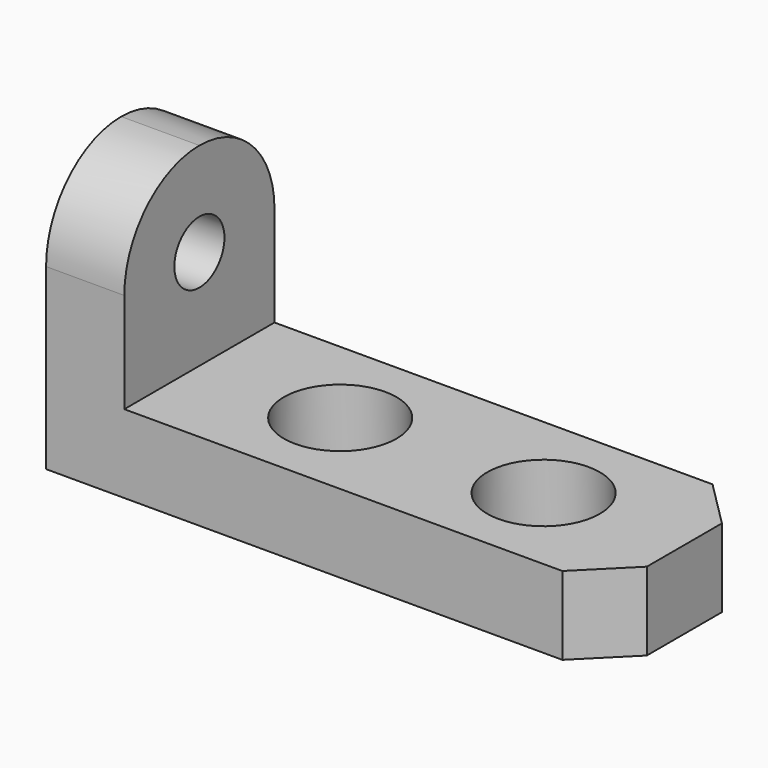
from build123d import *

# Parameters (mm, degrees)
F0_W     = 4572
F0_H     = 1524
F1_DEPTH = 635
F2_W     = 635
F2_H     = 1524
F3_DEPTH = 1574.8
F4_R     = 761.99999
F5_R     = 457.2
F6_DEPTH = 2540
F7_R     = 254
F8_DEPTH = 635
F9_SIZE  = 381


# Not quite as in the source:
# - a fillet or chamfer is up to 0.001 mm smaller than in the source, because OpenCascade refuses the exact size


with BuildPart() as f1:
    # F0 (on Top) → F1 (new body)
    with BuildSketch(Plane.XY):
        with Locations((2286, 762)):
            Rectangle(F0_W, F0_H)
    extrude(amount=F1_DEPTH)

    # F2 (on face) → F3 (join)
    with BuildSketch(Plane.XY.offset(635)):
        with Locations((317.5, 762)):
            Rectangle(F2_W, F2_H)
    extrude(amount=F3_DEPTH)

    # F4 (radius 762 in the source; OpenCascade refuses exactly that, so slightly less here)
    f4_edges = [f1.edges().sort_by_distance(p)[0] for p in [
        (317.5, 0, 2209.8),
        (317.5, 1524, 2209.8),
    ]]
    fillet(f4_edges, radius=F4_R)

    # F5 (on face) → F6 (cut)
    with BuildSketch(Plane.XY.offset(635)):
        with Locations((1778, 762)):
            Circle(F5_R)
        with Locations((3429, 762)):
            Circle(F5_R)
    extrude(amount=-F6_DEPTH, mode=Mode.SUBTRACT)

    # F7 (on face) → F8 (cut, through all)
    with BuildSketch(Plane.YZ.offset(635)):
        with Locations((762, 1447.8)):
            Circle(F7_R)
    extrude(amount=-F8_DEPTH, mode=Mode.SUBTRACT)

    # F9
    f9_edges = [f1.edges().sort_by_distance(p)[0] for p in [
        (4572, 0, 317.5),
        (4572, 1524, 317.5),
    ]]
    chamfer(f9_edges, length=F9_SIZE)


solid = f1.part
